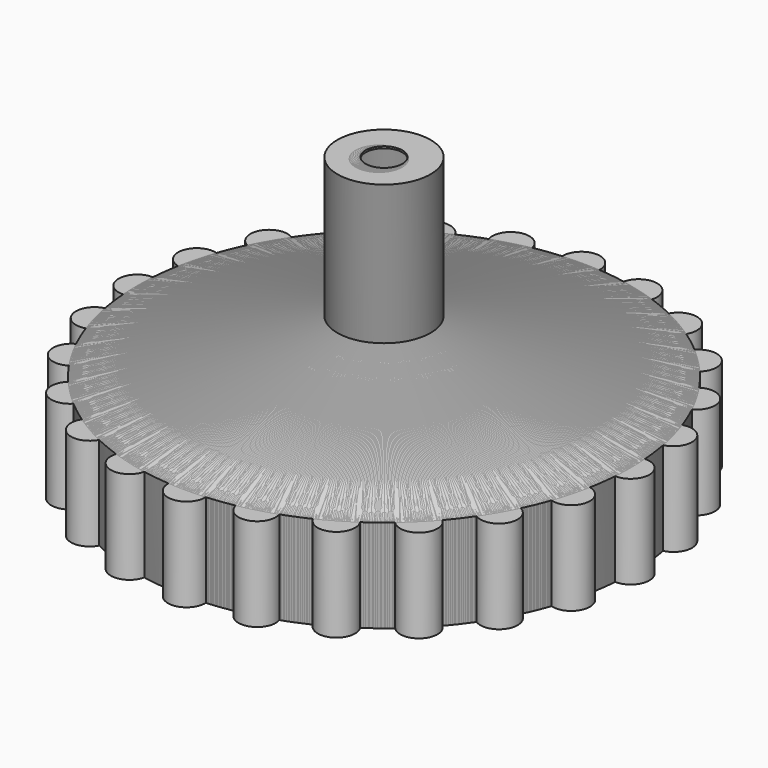
from build123d import *

# Parameters (mm, degrees)
F2_T     = -5.08
F3_R     = 63.5
F4_DEPTH = 781.3280539866
F6_DEPTH = 254
F7_COUNT = 24


with BuildPart() as f1:
    # F0 (on Front) → F1 (revolve)
    with BuildSketch(Plane.XZ):
        Polygon((-673.1, 254), (-673.1, 0), (0, 0), (0, 781.3270539866), (-127, 781.3270539866), (-127, 400.3270539866), align=None)
    revolve(axis=Axis((0, 0, 440.1198327541), (0, 0, 1)))

    # F2
    f2_openings = [f1.faces().sort_by_distance(p)[0] for p in [
        (0, 0, 0),
    ]]
    offset(amount=F2_T, openings=f2_openings, kind=Kind.INTERSECTION)

    # F3 (on face) → F4 (cut, through all)
    with BuildSketch(Plane.XY.offset(781.3270539866)):
        with Locations((0, -13.410911366)):
            Circle(F3_R)
    extrude(amount=-F4_DEPTH, mode=Mode.SUBTRACT)

    # F5 (on face) → F6 (join)
    with BuildSketch(Plane(origin=(0, 0, 0), x_dir=(1, 0, 0), z_dir=(0, 0, -1))):
        with BuildLine():
            ThreePointArc((673.1, 0), (672.6205839848, -25.4), (671.1830188679, -50.7638176592))
            ThreePointArc((671.1830188679, -50.7638176592), (723.9, 0), (671.1830188679, 50.7638176592))
            ThreePointArc((671.1830188679, 50.7638176592), (672.6205839848, 25.4), (673.1, 0))
        make_face()
    extrude(amount=-F6_DEPTH)


with BuildPart() as f7_1:
    # F7: instance of F1
    add(f1.part.rotate(Axis((0, 0, 781.3270539866), (0, 0, 1)), 1 * 360 / F7_COUNT))


with BuildPart() as f7_2:
    # F7: instance of F1
    add(f1.part.rotate(Axis((0, 0, 781.3270539866), (0, 0, 1)), 2 * 360 / F7_COUNT))


with BuildPart() as f7_3:
    # F7: instance of F1
    add(f1.part.rotate(Axis((0, 0, 781.3270539866), (0, 0, 1)), 3 * 360 / F7_COUNT))


with BuildPart() as f7_4:
    # F7: instance of F1
    add(f1.part.rotate(Axis((0, 0, 781.3270539866), (0, 0, 1)), 4 * 360 / F7_COUNT))


with BuildPart() as f7_5:
    # F7: instance of F1
    add(f1.part.rotate(Axis((0, 0, 781.3270539866), (0, 0, 1)), 5 * 360 / F7_COUNT))


with BuildPart() as f7_6:
    # F7: instance of F1
    add(f1.part.rotate(Axis((0, 0, 781.3270539866), (0, 0, 1)), 6 * 360 / F7_COUNT))


with BuildPart() as f7_7:
    # F7: instance of F1
    add(f1.part.rotate(Axis((0, 0, 781.3270539866), (0, 0, 1)), 7 * 360 / F7_COUNT))


with BuildPart() as f7_8:
    # F7: instance of F1
    add(f1.part.rotate(Axis((0, 0, 781.3270539866), (0, 0, 1)), 8 * 360 / F7_COUNT))


with BuildPart() as f7_9:
    # F7: instance of F1
    add(f1.part.rotate(Axis((0, 0, 781.3270539866), (0, 0, 1)), 9 * 360 / F7_COUNT))


with BuildPart() as f7_10:
    # F7: instance of F1
    add(f1.part.rotate(Axis((0, 0, 781.3270539866), (0, 0, 1)), 10 * 360 / F7_COUNT))


with BuildPart() as f7_11:
    # F7: instance of F1
    add(f1.part.rotate(Axis((0, 0, 781.3270539866), (0, 0, 1)), 11 * 360 / F7_COUNT))


with BuildPart() as f7_12:
    # F7: instance of F1
    add(f1.part.rotate(Axis((0, 0, 781.3270539866), (0, 0, 1)), 12 * 360 / F7_COUNT))


with BuildPart() as f7_13:
    # F7: instance of F1
    add(f1.part.rotate(Axis((0, 0, 781.3270539866), (0, 0, 1)), 13 * 360 / F7_COUNT))


with BuildPart() as f7_14:
    # F7: instance of F1
    add(f1.part.rotate(Axis((0, 0, 781.3270539866), (0, 0, 1)), 14 * 360 / F7_COUNT))


with BuildPart() as f7_15:
    # F7: instance of F1
    add(f1.part.rotate(Axis((0, 0, 781.3270539866), (0, 0, 1)), 15 * 360 / F7_COUNT))


with BuildPart() as f7_16:
    # F7: instance of F1
    add(f1.part.rotate(Axis((0, 0, 781.3270539866), (0, 0, 1)), 16 * 360 / F7_COUNT))


with BuildPart() as f7_17:
    # F7: instance of F1
    add(f1.part.rotate(Axis((0, 0, 781.3270539866), (0, 0, 1)), 17 * 360 / F7_COUNT))


with BuildPart() as f7_18:
    # F7: instance of F1
    add(f1.part.rotate(Axis((0, 0, 781.3270539866), (0, 0, 1)), 18 * 360 / F7_COUNT))


with BuildPart() as f7_19:
    # F7: instance of F1
    add(f1.part.rotate(Axis((0, 0, 781.3270539866), (0, 0, 1)), 19 * 360 / F7_COUNT))


with BuildPart() as f7_20:
    # F7: instance of F1
    add(f1.part.rotate(Axis((0, 0, 781.3270539866), (0, 0, 1)), 20 * 360 / F7_COUNT))


with BuildPart() as f7_21:
    # F7: instance of F1
    add(f1.part.rotate(Axis((0, 0, 781.3270539866), (0, 0, 1)), 21 * 360 / F7_COUNT))


with BuildPart() as f7_22:
    # F7: instance of F1
    add(f1.part.rotate(Axis((0, 0, 781.3270539866), (0, 0, 1)), 22 * 360 / F7_COUNT))


with BuildPart() as f7_23:
    # F7: instance of F1
    add(f1.part.rotate(Axis((0, 0, 781.3270539866), (0, 0, 1)), 23 * 360 / F7_COUNT))


solid = Compound([f1.part, f7_1.part, f7_2.part, f7_3.part, f7_4.part, f7_5.part, f7_6.part, f7_7.part, f7_8.part, f7_9.part, f7_10.part, f7_11.part, f7_12.part, f7_13.part, f7_14.part, f7_15.part, f7_16.part, f7_17.part, f7_18.part, f7_19.part, f7_20.part, f7_21.part, f7_22.part, f7_23.part])
